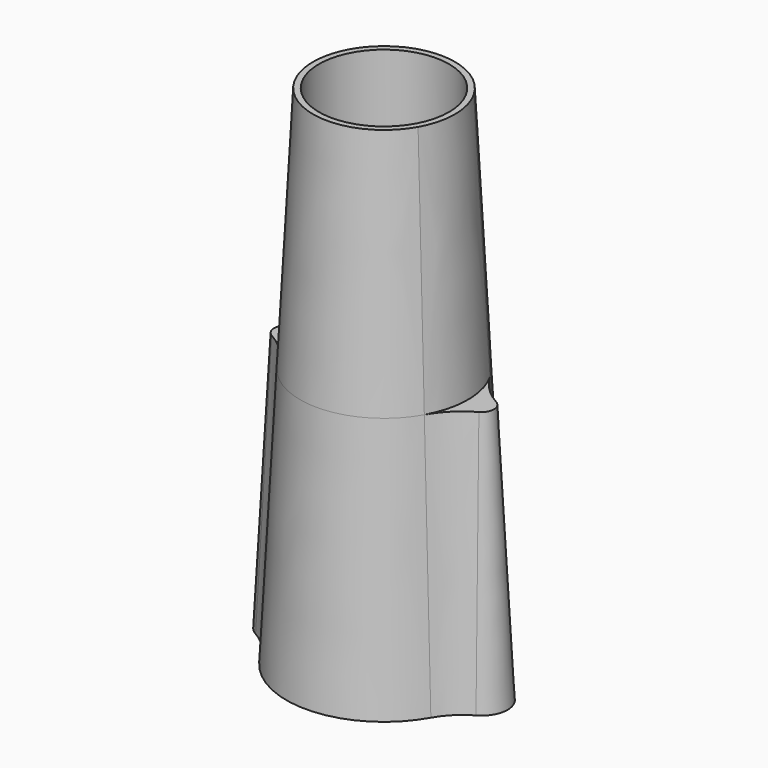
from build123d import *
from build123d import SkipClean  # not in build123d's __all__

# Parameters (mm, degrees)
F1_DEPTH = 20
F1_TAPER = 3
F3_DEPTH = 19
F3_TAPER = 3
F4_R     = 5
F5_DEPTH = 19
F6_R     = 4.5
F7_DEPTH = 20


with BuildPart() as f1:
    # F0 (on Top) → F1 (new body)
    with BuildSketch(Plane.XY):
        with BuildLine():
            ThreePointArc((-8.4714285714, -1.7482352618), (-7.3721516068, -2.5756206682), (-6.54, -3.6712940498))
            ThreePointArc((-6.54, -3.6712940498), (0, -7.5), (6.54, -3.6712940498))
            ThreePointArc((6.54, -3.6712940498), (7.3721516068, -2.5756206682), (8.4714285714, -1.7482352618))
            ThreePointArc((8.4714285714, -1.7482352618), (9.5, 0), (8.4714285714, 1.7482352618))
            ThreePointArc((8.4714285714, 1.7482352618), (7.3721516068, 2.5756206682), (6.54, 3.6712940498))
            ThreePointArc((6.54, 3.6712940498), (0, 7.5), (-6.54, 3.6712940498))
            ThreePointArc((-6.54, 3.6712940498), (-7.3721516068, 2.5756206682), (-8.4714285714, 1.7482352618))
            ThreePointArc((-8.4714285714, 1.7482352618), (-9.5, 0), (-8.4714285714, -1.7482352618))
        make_face()
    extrude(amount=F1_DEPTH, taper=F1_TAPER)

    # F2 (on face) → F3 (join)
    with BuildSketch(Plane.XY.offset(20)):
        with BuildLine():
            ThreePointArc((-5.6260083293, 3.1582157345), (-6.4518444143, 0), (-5.6260083293, -3.1582157345))
            ThreePointArc((-5.6260083293, -3.1582157345), (0, -6.4518444143), (5.6260083293, -3.1582157345))
            ThreePointArc((5.6260083293, -3.1582157345), (6.4518444143, 0), (5.6260083293, 3.1582157345))
            ThreePointArc((5.6260083293, 3.1582157345), (0, 6.4518444143), (-5.6260083293, 3.1582157345))
        make_face()
    with SkipClean():  # cleaning this boolean's faces spoils the solid; the shape is the same uncleaned
        extrude(amount=F3_DEPTH, taper=F3_TAPER)

    # F4 (on face) → F5 (cut)
    with BuildSketch(Plane.XY.offset(39)):
        Circle(F4_R)
    with SkipClean():  # cleaning this boolean's faces spoils the solid; the shape is the same uncleaned
        extrude(amount=-F5_DEPTH, mode=Mode.SUBTRACT)

    # F6 (on face) → F7 (cut, through all)
    with BuildSketch(Plane(origin=(0, 0, 0), x_dir=(1, 0, 0), z_dir=(0, 0, -1))):
        Circle(F6_R)
    with SkipClean():  # cleaning this boolean's faces spoils the solid; the shape is the same uncleaned
        extrude(amount=-F7_DEPTH, mode=Mode.SUBTRACT)


solid = f1.part
